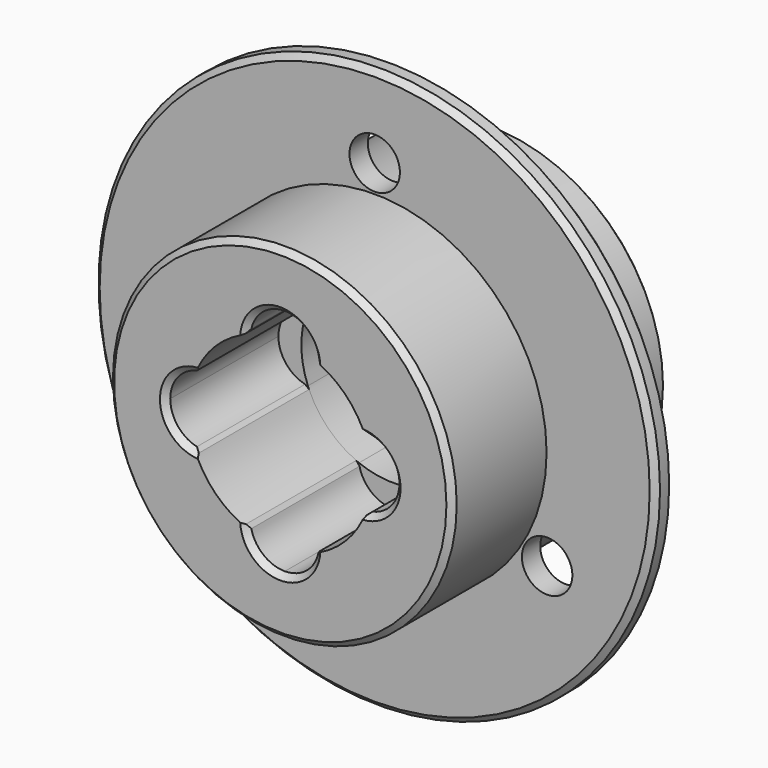
from build123d import *

# Parameters (mm, degrees)
F0_R          = 24.5
F0_R_2        = 1.5
F0_R_3        = 15
F1_DEPTH      = 2
F2_SIZE       = 0.5
F3_DEPTH      = 12.3
F4_SIZE       = 0.5
F6_R          = 8
F7_DEPTH      = 11.2
F9_DEPTH      = 23.501
F11_D         = 4.4
F6_R_2        = 15
F13_DEPTH     = 11.2
F14_T1_DEPTH  = 12.9973658511
F14_T6_ANGLE  = 212.7543214372
F14_T8_ANGLE  = 212.7543214372
F14_T10_ANGLE = 212.7543214371
F14_T12_ANGLE = 212.7543214372


# Not quite as in the source:
# - a fillet or chamfer that OpenCascade refuses, or shapes differently, is made with other operations: its cross-section is extruded or revolved along the edge and cut away or added
# - a feature of the source that left no trace in its solid (it failed there, or was rolled back) is left out


with BuildPart() as f1:
    # F0 (on Front) → F1 (new body)
    with BuildSketch(Plane.XZ):
        Circle(F0_R)
        with Locations((-15.0471913908, -8.6875)):
            Circle(F0_R_2, mode=Mode.SUBTRACT)
        Circle(F0_R_3, mode=Mode.SUBTRACT)
        with Locations((15.0471913908, -8.6875)):
            Circle(F0_R_2, mode=Mode.SUBTRACT)
        with Locations((0, 17.375)):
            Circle(F0_R_2, mode=Mode.SUBTRACT)
    extrude(amount=F1_DEPTH)

    # F2
    f2_edges = [f1.edges().sort_by_distance(p)[0] for p in [
        (-24.5, -2, 0),
        (-24.5, 0, 0),
    ]]
    chamfer(f2_edges, length=F2_SIZE)

    # F0 (on Front) → F3 (join)
    with BuildSketch(Plane.XZ):
        Circle(F0_R_3)
        with Locations((0, 17.375)):
            Circle(F0_R_2)
        with Locations((15.0471913908, -8.6875)):
            Circle(F0_R_2)
        with Locations((-15.0471913908, -8.6875)):
            Circle(F0_R_2)
    extrude(amount=F3_DEPTH)

    # F4
    f4_edges = [f1.edges().sort_by_distance(p)[0] for p in [
        (-15, -12.3, 0),
    ]]
    chamfer(f4_edges, length=F4_SIZE)

    # F6 (on face) → F7 (join)
    with BuildSketch(Plane.XZ):
        Circle(F6_R)
    extrude(amount=-F7_DEPTH)

    # F5 (on face) → F9 (cut, through all)
    with BuildSketch(Plane.XZ.offset(12.3)):
        with BuildLine():
            ThreePointArc((7.4285714286, -2.9692299558), (7.8558440485, -1.511857892), (8, 0))
            ThreePointArc((8, 0), (7.8558440485, 1.511857892), (7.4285714286, 2.9692299558))
            ThreePointArc((7.4285714286, 2.9692299558), (5.6568542495, 5.6568542495), (2.9692299558, 7.4285714286))
            ThreePointArc((2.9692299558, 7.4285714286), (0, 8), (-2.9692299558, 7.4285714286))
            ThreePointArc((-2.9692299558, 7.4285714286), (-5.6568542495, 5.6568542495), (-7.4285714286, 2.9692299558))
            ThreePointArc((-7.4285714286, 2.9692299558), (-8, 0), (-7.4285714286, -2.9692299558))
            ThreePointArc((-7.4285714286, -2.9692299558), (-5.6568542495, -5.6568542495), (-2.9692299558, -7.4285714286))
            ThreePointArc((-2.9692299558, -7.4285714286), (0, -8), (2.9692299558, -7.4285714286))
            ThreePointArc((2.9692299558, -7.4285714286), (5.6568542495, -5.6568542495), (7.4285714286, -2.9692299558))
        make_face()
        with BuildLine():
            ThreePointArc((-2.9692299558, 7.4285714286), (0, 8), (2.9692299558, 7.4285714286))
            ThreePointArc((2.9692299558, 7.4285714286), (1.9639610121, 9.2677868381), (0, 10))
            ThreePointArc((0, 10), (-1.9639610121, 9.2677868381), (-2.9692299558, 7.4285714286))
        make_face()
        with BuildLine():
            ThreePointArc((-7.4285714286, -2.9692299558), (-8, 0), (-7.4285714286, 2.9692299558))
            ThreePointArc((-7.4285714286, 2.9692299558), (-9.2677868381, 1.9639610121), (-10, 0))
            ThreePointArc((-10, 0), (-9.2677868381, -1.9639610121), (-7.4285714286, -2.9692299558))
        make_face()
        with BuildLine():
            ThreePointArc((7.4285714286, 2.9692299558), (7.8558440485, 1.511857892), (8, 0))
            ThreePointArc((8, 0), (7.8558440485, -1.511857892), (7.4285714286, -2.9692299558))
            ThreePointArc((7.4285714286, -2.9692299558), (9.2677868381, -1.9639610121), (10, 0))
            ThreePointArc((10, 0), (9.2677868381, 1.9639610121), (7.4285714286, 2.9692299558))
        make_face()
        with BuildLine():
            ThreePointArc((0, -10), (1.9639610121, -9.2677868381), (2.9692299558, -7.4285714286))
            ThreePointArc((2.9692299558, -7.4285714286), (0, -8), (-2.9692299558, -7.4285714286))
            ThreePointArc((-2.9692299558, -7.4285714286), (-1.9639610121, -9.2677868381), (0, -10))
        make_face()
    extrude(amount=-F9_DEPTH, mode=Mode.SUBTRACT)

    # F11 (through all)
    with Locations(Plane(origin=(0, 0, 0), x_dir=(1, 0, 0), z_dir=(0, 1, 0))):
        with Locations((0, -17.375), (15.0471913908, 8.6875), (-15.0471913908, 8.6875)):
            Hole(F11_D / 2)

    # F12 (on face) + F6 (on face) → F13 (join)
    with BuildSketch(Plane(origin=(0, 0, 0), x_dir=(-1, 0, 0), z_dir=(0, 1, 0))):
        with BuildLine():
            ThreePointArc((10, 0), (9.2677868381, -1.9639610121), (7.4285714286, -2.9692299558))
            ThreePointArc((7.4285714286, -2.9692299558), (5.6568542495, -5.6568542495), (2.9692299558, -7.4285714286))
            ThreePointArc((2.9692299558, -7.4285714286), (1.9639610121, -9.2677868381), (0, -10))
            ThreePointArc((0, -10), (7.0710678119, -7.0710678119), (10, 0))
        make_face()
        with BuildLine():
            ThreePointArc((-10, 0), (-7.0710678119, -7.0710678119), (0, -10))
            ThreePointArc((0, -10), (-1.9639610121, -9.2677868381), (-2.9692299558, -7.4285714286))
            ThreePointArc((-2.9692299558, -7.4285714286), (-5.6568542495, -5.6568542495), (-7.4285714286, -2.9692299558))
            ThreePointArc((-7.4285714286, -2.9692299558), (-9.2677868381, -1.9639610121), (-10, 0))
        make_face()
        with BuildLine():
            ThreePointArc((2.9692299558, 7.4285714286), (5.6568542495, 5.6568542495), (7.4285714286, 2.9692299558))
            ThreePointArc((7.4285714286, 2.9692299558), (9.2677868381, 1.9639610121), (10, 0))
            ThreePointArc((10, 0), (7.0710678119, 7.0710678119), (0, 10))
            ThreePointArc((0, 10), (1.9639610121, 9.2677868381), (2.9692299558, 7.4285714286))
        make_face()
    with BuildSketch(Plane.XZ):
        Circle(F6_R_2)
        Circle(F6_R, mode=Mode.SUBTRACT)
    extrude(amount=F13_DEPTH, dir=(0, 1, 0))

    # F14: chamfer of 0.5 on 13 edges, made by hand

    # F14_s2 → F14_t1 (cut)
    with BuildSketch(Plane.XZ):
        with BuildLine():
            Line((-3.2228041391, 7.3123337651), (-2.9106652166, 7.6888667151))
            Line((-2.9106652166, 7.6888667151), (-2.9009204522, 7.6866218171))
            ThreePointArc((-2.9009204522, 7.6866218171), (-2.9374254667, 7.5582397584), (-2.9593325226, 7.4271428571))
            Line((-2.9593325226, 7.4271428571), (-2.9655184184, 7.4192857143))
            ThreePointArc((-2.9655184184, 7.4192857143), (-3.0943502859, 7.3664846642), (-3.2187915891, 7.3031741013))
            Line((-3.2187915891, 7.3031741013), (-3.2228041391, 7.3123337651))
        make_face()
        with BuildLine():
            Line((7.3123337651, -3.2228041391), (7.6888667151, -2.9106652166))
            Line((7.6888667151, -2.9106652166), (7.6866218171, -2.9009204522))
            ThreePointArc((7.6866218171, -2.9009204522), (7.5582397584, -2.9374254667), (7.4271428571, -2.9593325226))
            Line((7.4271428571, -2.9593325226), (7.4192857143, -2.9655184184))
            ThreePointArc((7.4192857143, -2.9655184184), (7.3664846642, -3.0943502859), (7.3031741013, -3.2187915891))
            Line((7.3031741013, -3.2187915891), (7.3123337651, -3.2228041391))
        make_face()
        with BuildLine():
            Line((3.2228041391, -7.3123337651), (2.9106652166, -7.6888667151))
            Line((2.9106652166, -7.6888667151), (2.9009204522, -7.6866218171))
            ThreePointArc((2.9009204522, -7.6866218171), (2.9374254667, -7.5582397584), (2.9593325226, -7.4271428571))
            Line((2.9593325226, -7.4271428571), (2.9655184184, -7.4192857143))
            ThreePointArc((2.9655184184, -7.4192857143), (3.0943502859, -7.3664846642), (3.2187915891, -7.3031741013))
            Line((3.2187915891, -7.3031741013), (3.2228041391, -7.3123337651))
        make_face()
        with BuildLine():
            Line((-3.2228041391, -7.3123337651), (-2.9106652166, -7.6888667151))
            Line((-2.9106652166, -7.6888667151), (-2.9009204522, -7.6866218171))
            ThreePointArc((-2.9009204522, -7.6866218171), (-2.9374254667, -7.5582397584), (-2.9593325226, -7.4271428571))
            Line((-2.9593325226, -7.4271428571), (-2.9655184184, -7.4192857143))
            ThreePointArc((-2.9655184184, -7.4192857143), (-3.0943502859, -7.3664846642), (-3.2187915891, -7.3031741013))
            Line((-3.2187915891, -7.3031741013), (-3.2228041391, -7.3123337651))
        make_face()
        with BuildLine():
            Line((-7.3123337651, -3.2228041391), (-7.6888667151, -2.9106652166))
            Line((-7.6888667151, -2.9106652166), (-7.6866218171, -2.9009204522))
            ThreePointArc((-7.6866218171, -2.9009204522), (-7.5582397584, -2.9374254667), (-7.4271428571, -2.9593325226))
            Line((-7.4271428571, -2.9593325226), (-7.4192857143, -2.9655184184))
            ThreePointArc((-7.4192857143, -2.9655184184), (-7.3664846642, -3.0943502859), (-7.3031741013, -3.2187915891))
            Line((-7.3031741013, -3.2187915891), (-7.3123337651, -3.2228041391))
        make_face()
        with BuildLine():
            Line((-7.3123337651, 3.2228041391), (-7.6888667151, 2.9106652166))
            Line((-7.6888667151, 2.9106652166), (-7.6866218171, 2.9009204522))
            ThreePointArc((-7.6866218171, 2.9009204522), (-7.5582397584, 2.9374254667), (-7.4271428571, 2.9593325226))
            Line((-7.4271428571, 2.9593325226), (-7.4192857143, 2.9655184184))
            ThreePointArc((-7.4192857143, 2.9655184184), (-7.3664846642, 3.0943502859), (-7.3031741013, 3.2187915891))
            Line((-7.3031741013, 3.2187915891), (-7.3123337651, 3.2228041391))
        make_face()
        with BuildLine():
            Line((7.6888667151, 2.9106652166), (7.3123337651, 3.2228041391))
            Line((7.3123337651, 3.2228041391), (7.3031741013, 3.2187915891))
            ThreePointArc((7.3031741013, 3.2187915891), (7.3664846642, 3.0943502859), (7.4192857143, 2.9655184184))
            Line((7.4192857143, 2.9655184184), (7.4271428571, 2.9593325226))
            ThreePointArc((7.4271428571, 2.9593325226), (7.5582397584, 2.9374254667), (7.6866218171, 2.9009204522))
            Line((7.6866218171, 2.9009204522), (7.6888667151, 2.9106652166))
        make_face()
        with BuildLine():
            Line((3.2228041391, 7.3123337651), (2.9106652166, 7.6888667151))
            Line((2.9106652166, 7.6888667151), (2.9009204522, 7.6866218171))
            ThreePointArc((2.9009204522, 7.6866218171), (2.9374254667, 7.5582397584), (2.9593325226, 7.4271428571))
            Line((2.9593325226, 7.4271428571), (2.9655184184, 7.4192857143))
            ThreePointArc((2.9655184184, 7.4192857143), (3.0943502859, 7.3664846642), (3.2187915891, 7.3031741013))
            Line((3.2187915891, 7.3031741013), (3.2228041391, 7.3123337651))
        make_face()
    extrude(amount=F14_T1_DEPTH, mode=Mode.SUBTRACT)

    # F14_s3 → F14_t4 (revolve, cut)
    with BuildSketch(Plane.XY):
        with BuildLine():
            Line((15.0141421356, 10.6858578644), (14.4858578644, 11.2141421356))
            Line((14.4858578644, 11.2141421356), (14.4858578644, 11.2241421356))
            ThreePointArc((14.4858578644, 11.2241421356), (14.7429289322, 11.21), (15, 11.21))
            Line((15, 11.21), (15.01, 11.2))
            ThreePointArc((15.01, 11.2), (15.01, 10.9429289322), (15.0241421356, 10.6858578644))
            Line((15.0241421356, 10.6858578644), (15.0141421356, 10.6858578644))
        make_face()
    revolve(axis=Axis((0, 11.2, 0), (0, -1, 0)), mode=Mode.SUBTRACT)

    # F14_s5 → F14_t6 (revolve, cut)
    with BuildSketch(Plane(origin=(-6.4434937297, 0, 1.8936326632), x_dir=(0, 1, 0), z_dir=(0.9594264455, 0, -0.2819590321))):
        with BuildLine():
            Line((-11.7858578644, 1.01214464), (-12.3141421356, 1.5404289113))
            Line((-12.3141421356, 1.5404289113), (-12.3241421356, 1.5404289113))
            ThreePointArc((-12.3241421356, 1.5404289113), (-12.31, 1.2833578434), (-12.31, 1.0262867756))
            Line((-12.31, 1.0262867756), (-12.3, 1.0162867756))
            ThreePointArc((-12.3, 1.0162867756), (-12.0429289322, 1.0162867756), (-11.7858578644, 1.00214464))
            Line((-11.7858578644, 1.00214464), (-11.7858578644, 1.01214464))
        make_face()
    revolve(axis=Axis((-7, -12.3, 0), (0, -1, 0)), revolution_arc=F14_T6_ANGLE, mode=Mode.SUBTRACT)

    # F14_s7 → F14_t8 (revolve, cut)
    with BuildSketch(Plane(origin=(-1.8936326632, 0, -6.4434937297), x_dir=(0, 1, 0), z_dir=(0.2819590321, 0, 0.9594264455))):
        with BuildLine():
            Line((-11.7858578644, 1.01214464), (-12.3141421356, 1.5404289113))
            Line((-12.3141421356, 1.5404289113), (-12.3241421356, 1.5404289113))
            ThreePointArc((-12.3241421356, 1.5404289113), (-12.31, 1.2833578434), (-12.31, 1.0262867756))
            Line((-12.31, 1.0262867756), (-12.3, 1.0162867756))
            ThreePointArc((-12.3, 1.0162867756), (-12.0429289322, 1.0162867756), (-11.7858578644, 1.00214464))
            Line((-11.7858578644, 1.00214464), (-11.7858578644, 1.01214464))
        make_face()
    revolve(axis=Axis((0, -12.3, -7), (0, -1, 0)), revolution_arc=F14_T8_ANGLE, mode=Mode.SUBTRACT)

    # F14_s9 → F14_t10 (revolve, cut)
    with BuildSketch(Plane(origin=(6.4434937297, 0, -1.8936326632), x_dir=(0, 1, 0), z_dir=(-0.9594264455, 0, 0.2819590321))):
        with BuildLine():
            Line((-11.7858578644, 1.01214464), (-12.3141421356, 1.5404289113))
            Line((-12.3141421356, 1.5404289113), (-12.3241421356, 1.5404289113))
            ThreePointArc((-12.3241421356, 1.5404289113), (-12.31, 1.2833578434), (-12.31, 1.0262867756))
            Line((-12.31, 1.0262867756), (-12.3, 1.0162867756))
            ThreePointArc((-12.3, 1.0162867756), (-12.0429289322, 1.0162867756), (-11.7858578644, 1.00214464))
            Line((-11.7858578644, 1.00214464), (-11.7858578644, 1.01214464))
        make_face()
    revolve(axis=Axis((7, -12.3, 0), (0, -1, 0)), revolution_arc=F14_T10_ANGLE, mode=Mode.SUBTRACT)

    # F14_s11 → F14_t12 (revolve, cut)
    with BuildSketch(Plane(origin=(1.8936326632, 0, 6.4434937297), x_dir=(0, 1, 0), z_dir=(-0.2819590321, 0, -0.9594264455))):
        with BuildLine():
            Line((-11.7858578644, 1.01214464), (-12.3141421356, 1.5404289113))
            Line((-12.3141421356, 1.5404289113), (-12.3241421356, 1.5404289113))
            ThreePointArc((-12.3241421356, 1.5404289113), (-12.31, 1.2833578434), (-12.31, 1.0262867756))
            Line((-12.31, 1.0262867756), (-12.3, 1.0162867756))
            ThreePointArc((-12.3, 1.0162867756), (-12.0429289322, 1.0162867756), (-11.7858578644, 1.00214464))
            Line((-11.7858578644, 1.00214464), (-11.7858578644, 1.01214464))
        make_face()
    revolve(axis=Axis((0, -12.3, 7), (0, -1, 0)), revolution_arc=F14_T12_ANGLE, mode=Mode.SUBTRACT)


solid = f1.part
